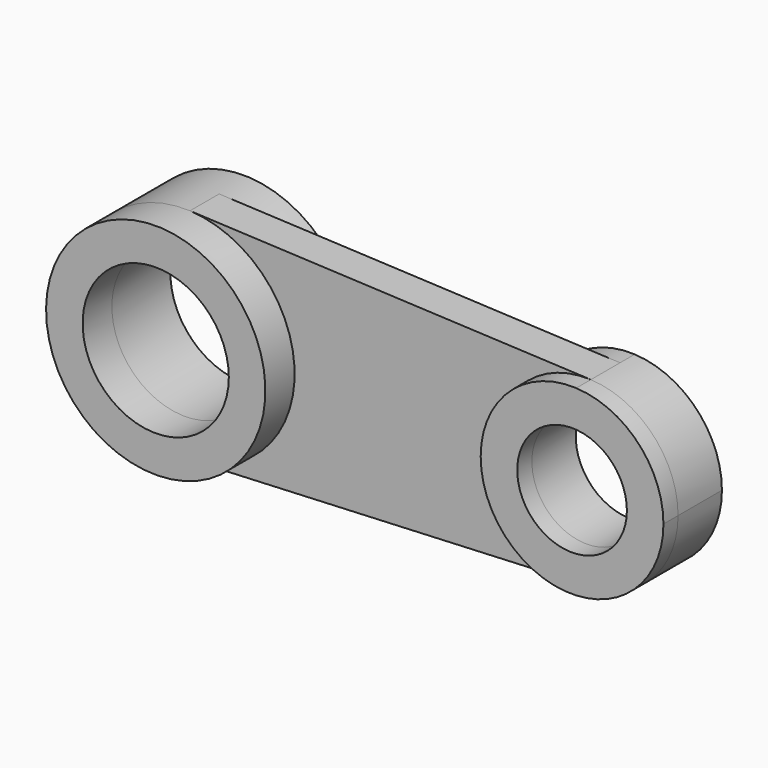
from build123d import *

# Parameters (mm, degrees)
F1_DEPTH = 10
F0_R     = 20
F2_DEPTH = 20
F0_R_2   = 15
F3_DEPTH = 15
F4_DEPTH = 10
F5_DEPTH = 5


with BuildPart() as f1:
    # F0 (on Front) → F1 (new body)
    with BuildSketch(Plane.XZ):
        with BuildLine():
            ThreePointArc((-67.8919983579, 29.9689394462), (-47.5664292993, 20.7250586992), (-39.2567944856, 0))
            ThreePointArc((-39.2567944856, 0), (-47.5664292993, -20.7250586992), (-67.8919983579, -29.9689394462))
            Line((-67.8919983579, -29.9689394462), (41.7870608186, -24.9741162052))
            ThreePointArc((41.7870608186, -24.9741162052), (15.6497307122, 0), (41.7870608186, 24.9741162052))
            Line((41.7870608186, 24.9741162052), (-67.8919983579, 29.9689394462))
        make_face()
    extrude(amount=-F1_DEPTH)

    # F0 (on Front) → F2 (join)
    with BuildSketch(Plane.XZ):
        with BuildLine():
            ThreePointArc((-67.8919983579, -29.9689394462), (-47.5664292993, -20.7250586992), (-39.2567944856, 0))
            ThreePointArc((-39.2567944856, 0), (-47.5664292993, 20.7250586992), (-67.8919983579, 29.9689394462))
            ThreePointArc((-67.8919983579, 29.9689394462), (-99.2567944856, 0), (-67.8919983579, -29.9689394462))
        make_face()
        with Locations((-69.2567944856, 0)):
            Circle(F0_R, mode=Mode.SUBTRACT)
    extrude(amount=-F2_DEPTH)

    # F0 (on Front) → F4 (join)
    with BuildSketch(Plane.XZ):
        with BuildLine():
            ThreePointArc((-67.8919983579, -29.9689394462), (-47.5664292993, -20.7250586992), (-39.2567944856, 0))
            ThreePointArc((-39.2567944856, 0), (-47.5664292993, 20.7250586992), (-67.8919983579, 29.9689394462))
            ThreePointArc((-67.8919983579, 29.9689394462), (-99.2567944856, 0), (-67.8919983579, -29.9689394462))
        make_face()
        with Locations((-69.2567944856, 0)):
            Circle(F0_R, mode=Mode.SUBTRACT)
    extrude(amount=F4_DEPTH)


with BuildPart() as f3:
    # F0 (on Front) → F3 (new body)
    with BuildSketch(Plane.XZ):
        with BuildLine():
            ThreePointArc((65.6497307122, 0), (58.7250350341, 17.2708822493), (41.7870608186, 24.9741162052))
            ThreePointArc((41.7870608186, 24.9741162052), (15.6497307122, 0), (41.7870608186, -24.9741162052))
            ThreePointArc((41.7870608186, -24.9741162052), (58.7250350341, -17.2708822493), (65.6497307122, 0))
        make_face()
        with Locations((40.6497307122, 0)):
            Circle(F0_R_2, mode=Mode.SUBTRACT)
    extrude(amount=-F3_DEPTH)

    # F0 (on Front) → F5 (join)
    with BuildSketch(Plane.XZ):
        with BuildLine():
            ThreePointArc((65.6497307122, 0), (58.7250350341, 17.2708822493), (41.7870608186, 24.9741162052))
            ThreePointArc((41.7870608186, 24.9741162052), (15.6497307122, 0), (41.7870608186, -24.9741162052))
            ThreePointArc((41.7870608186, -24.9741162052), (58.7250350341, -17.2708822493), (65.6497307122, 0))
        make_face()
        with Locations((40.6497307122, 0)):
            Circle(F0_R_2, mode=Mode.SUBTRACT)
    extrude(amount=F5_DEPTH)


solid = Compound([f1.part, f3.part])
